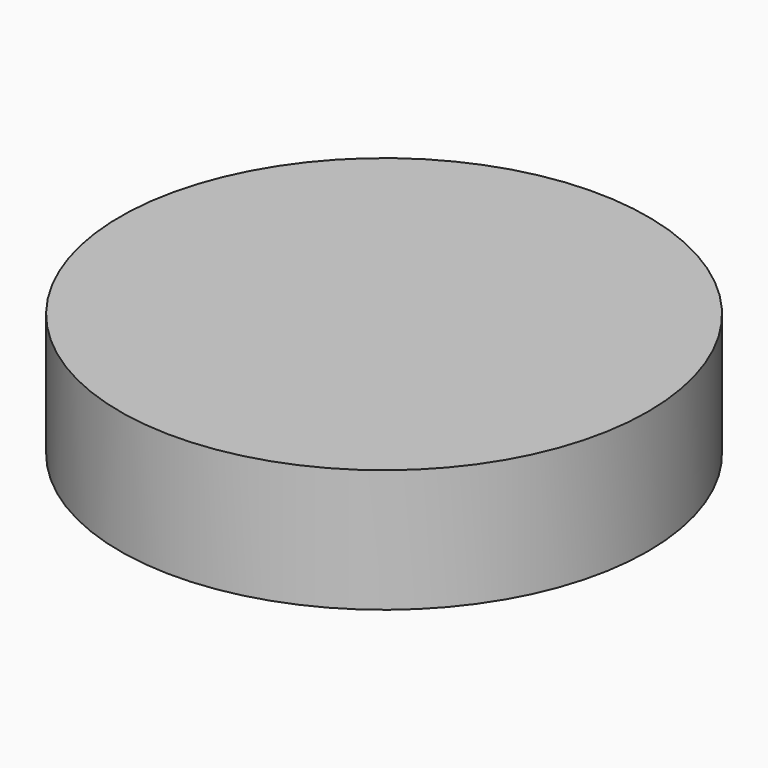
from build123d import *

# Parameters (mm, degrees)
F0_R     = 53.6968168664
F3_DEPTH = 25


# Not quite as in the source:
# - the program builds the solid bodies; features that only make, move or delete a surface that nothing else refers to are left out


with BuildPart() as f3:
    # F0 (on Top) → F3 (new body)
    with BuildSketch(Plane.XY):
        Circle(F0_R)
    extrude(amount=F3_DEPTH)


solid = f3.part
